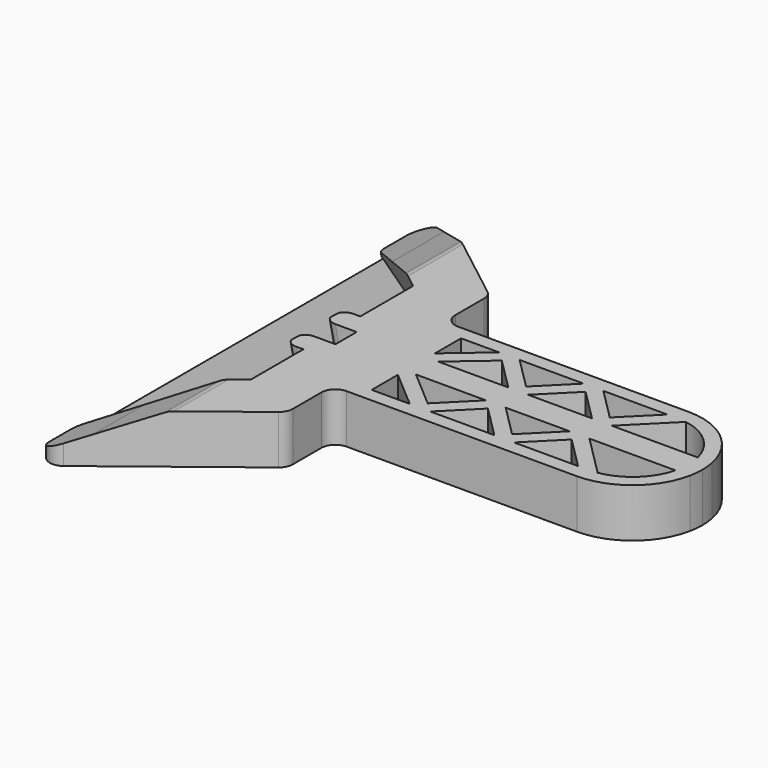
from build123d import *

# Parameters (mm, degrees)
F1_DEPTH      = 7
F5_DEPTH      = 0.8
F6_REACH      = 40.8395042988
F7_W          = 36.7298226772
F7_H          = 7
F8_DEPTH      = 1
F9_DEPTH      = 45
F10_T1_DEPTH  = 7
F10_T3_DEPTH  = 21.8461795352
F10_T5_DEPTH  = 11.8964874596
F10_T7_DEPTH  = 11.956767541
F10_T12_DEPTH = 5.3023503656


# Not quite as in the source:
# - a fillet or chamfer that OpenCascade refuses, or shapes differently, is made with other operations: its cross-section is extruded or revolved along the edge and cut away or added


with BuildPart() as f1:
    # F0 (on Top) → F1 (new body)
    with BuildSketch(Plane.XY):
        with BuildLine():
            Line((0, 0), (0, -36.7298226772))
            Line((0, -36.7298226772), (24, -18.0982437298))
            Line((24, -18.0982437298), (24, -10))
            Line((24, -10), (59, -10))
            ThreePointArc((59, -10), (65.3245553203, -7.7459666924), (68.7979589711, -2))
            ThreePointArc((68.7979589711, -2), (68.9493615301, -1.0050896201), (69, 0))
            Line((69, 0), (0, 0))
        make_face()
        Polygon((33.4652661258, -8), (28.0146803707, -8), (28.0146803707, -3.3182508079), align=None, mode=Mode.SUBTRACT)
        Polygon((41, -3.4142135624), (45.5857864376, -8), (36.4142135624, -8), align=None, mode=Mode.SUBTRACT)
        Polygon((29.5494142449, -2), (39.5857864376, -2), (34.9483778196, -6.637408618), align=None, mode=Mode.SUBTRACT)
        Polygon((42.4142135624, -2), (51.5857864376, -2), (47, -6.5857864376), align=None, mode=Mode.SUBTRACT)
        Polygon((53, -3.4142135624), (57.5857864376, -8), (48.4142135624, -8), align=None, mode=Mode.SUBTRACT)
        with BuildLine():
            ThreePointArc((66.7459666924, -2), (64.4007894962, -5.9018194498), (60.3067648391, -7.8925512767))
            Line((60.3067648391, -7.8925512767), (54.4142135624, -2))
            Line((54.4142135624, -2), (66.7459666924, -2))
        make_face(mode=Mode.SUBTRACT)
    extrude(amount=F1_DEPTH)

    # F4 (on face) → F5 (cut)
    with BuildSketch(Plane(origin=(0, 0, 0), x_dir=(0.9781476007, 0, 0.2079116908), z_dir=(0.2079116908, 0, -0.9781476007))):
        Polygon((19, 15.5), (0, 30.75), (0, 28.1854591432), (17, 14.5407223011), (17, 5.1), (19, 5.1), align=None)
        with BuildLine():
            Line((17, 14.5407223011), (0, 28.1854591432))
            Line((0, 28.1854591432), (0, 0))
            Line((0, 0), (19, 0))
            Line((19, 0), (19, 1.9))
            Line((19, 1.9), (16, 1.9))
            ThreePointArc((16, 1.9), (14.4, 3.5), (16, 5.1))
            Line((16, 5.1), (17, 5.1))
            Line((17, 5.1), (17, 14.5407223011))
        make_face()
    extrude(amount=-F5_DEPTH, mode=Mode.SUBTRACT)

    f6_end = Plane(origin=(20.8323918984, -11.3984937311, 7), x_dir=(1, 0, 0), z_dir=(0, 0, 1))
    # F4 (on face) → F6 (cut, up to a plane its end follows)
    with BuildSketch(Plane(origin=(0, 0, 0), x_dir=(0.9781476007, 0, 0.2079116908), z_dir=(0.2079116908, 0, -0.9781476007))):
        with BuildLine():
            Line((17, 14.5407223011), (0, 28.1854591432))
            Line((0, 28.1854591432), (0, 0))
            Line((0, 0), (19, 0))
            Line((19, 0), (19, 1.9))
            Line((19, 1.9), (16, 1.9))
            ThreePointArc((16, 1.9), (14.4, 3.5), (16, 5.1))
            Line((16, 5.1), (17, 5.1))
            Line((17, 5.1), (17, 14.5407223011))
        make_face()
    f6_long = extrude(amount=-F6_REACH, mode=Mode.PRIVATE)
    add(split(f6_long, bisect_by=f6_end, keep=Keep.BOTTOM, mode=Mode.PRIVATE), mode=Mode.SUBTRACT)

    # F7 (on face) → F8 (cut)
    with BuildSketch(Plane(origin=(0, 0, 0), x_dir=(0, -1, 0), z_dir=(-1, 0, 0))):
        with Locations((18.3649113386, 3.5)):
            Rectangle(F7_W, F7_H)
    extrude(amount=-F8_DEPTH, mode=Mode.SUBTRACT)

    # F2 (on face) → F9 (cut)
    with BuildSketch(Plane(origin=(0, 0, 0), x_dir=(-1, 0, 0), z_dir=(0, 1, 0))):
        Polygon((0, 4), (-6.7871916141, 4), (0, 0.9781476007), align=None)
        Polygon((-13.5253019358, 7), (-6.7871916141, 4), (0, 4), (0, 7), align=None)
    extrude(amount=-F9_DEPTH, mode=Mode.SUBTRACT)

    # F10: fillet of radius 2 on 5 edges, made by hand

    # F10_s2 → F10_t1 (join)
    with BuildSketch(Plane.XY):
        with BuildLine():
            ThreePointArc((24, -12), (24.5857864376, -10.5857864376), (26, -10))
            Line((26, -10), (24, -10))
            Line((24, -10), (24, -12))
        make_face()
    extrude(amount=F10_T1_DEPTH)

    # F10_s4 → F10_t3 (cut)
    with BuildSketch(Plane.XY.offset(-10.2114016246)):
        with BuildLine():
            ThreePointArc((4.2264416068, -33.4487693246), (2.1204783157, -33.6651760692), (1, -31.8689462379))
            Line((1, -31.8689462379), (1, -35.9535068877))
            Line((1, -35.9535068877), (4.2264416068, -33.4487693246))
        make_face()
    extrude(amount=F10_T3_DEPTH, mode=Mode.SUBTRACT)

    # F10_s6 → F10_t5 (cut)
    with BuildSketch(Plane.XY.offset(-2.4482437298)):
        with BuildLine():
            ThreePointArc((24, -17.1189462379), (23.7962298313, -17.9984679222), (23.2264416068, -18.6987693246))
            Line((23.2264416068, -18.6987693246), (24, -18.0982437298))
            Line((24, -18.0982437298), (24, -17.1189462379))
        make_face()
    extrude(amount=F10_T5_DEPTH, mode=Mode.SUBTRACT)

    # F10_s8 → F10_t7 (cut)
    with BuildSketch(Plane.XZ.offset(15.3359324944)):
        with BuildLine():
            ThreePointArc((13.9504150591, 7), (13.5345916775, 6.9562952015), (13.136941773, 6.8270909153))
            Line((13.136941773, 6.8270909153), (13.5253019358, 7))
            Line((13.5253019358, 7), (13.9504150591, 7))
        make_face()
    extrude(amount=F10_T7_DEPTH, mode=Mode.SUBTRACT)


with BuildPart() as f10_tool10:
    # F10_s11 → F10_t12 (new body)
    with BuildSketch(Plane(origin=(0, -0.1012401159, -0.6066769302), x_dir=(1, 0, 0), z_dir=(0, -0.1646003505, -0.9863603422))):
        with BuildLine():
            ThreePointArc((1, 28.0074292273), (1.2043011265, 27.126824006), (1.7754655557, 26.4261274235))
            Line((1.7754655557, 26.4261274235), (1, 27.0266353601))
            Line((1, 27.0266353601), (1, 28.0074292273))
        make_face()
    extrude(amount=F10_T12_DEPTH)

    split(bisect_by=Plane(origin=(-0.1663293527, 0, 0.7825180806), x_dir=(0, 1, 0), z_dir=(-0.2079116908, 0, 0.9781476007)), keep=Keep.TOP)


with BuildPart() as f1_1:
    add(f1.part)

    # F10_t9: cut F10_tool10
    add(f10_tool10.part, mode=Mode.SUBTRACT)

    # F11: F1 across plane


with BuildPart() as f1_2:
    add(f1_1.part)
    add(f1_1.part.mirror(Plane.XZ))


solid = f1_2.part
